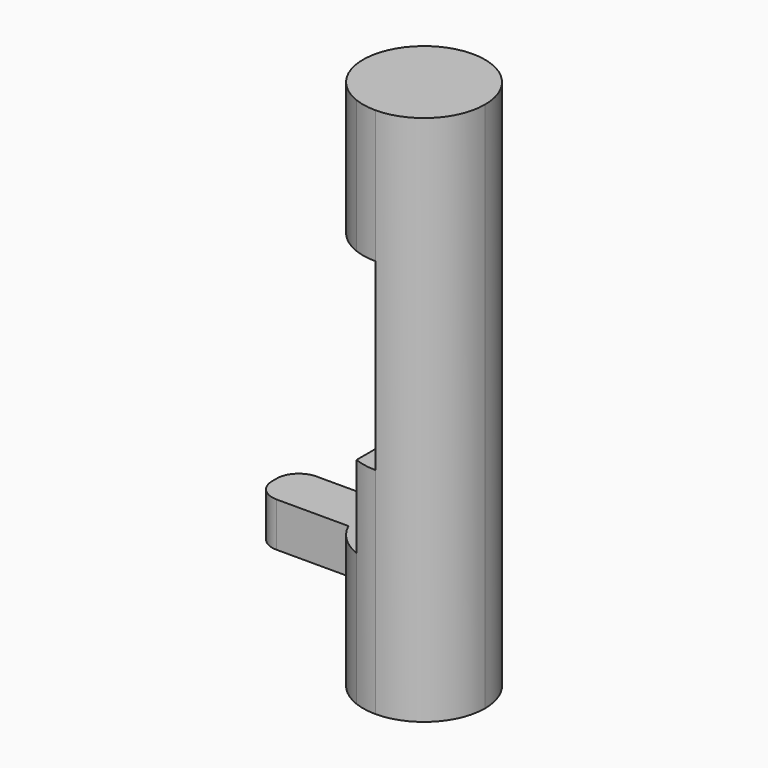
from build123d import *
from build123d import SkipClean  # not in build123d's __all__

# Parameters (mm, degrees)
F1_DEPTH = 24
F2_DEPTH = 18
F3_DEPTH = 9.7
F4_DEPTH = 6
F5_DEPTH = 6
F6_R     = 1
F7_DEPTH = 4


with BuildPart() as f1:
    # F0 (on Top) → F1 (new body)
    with BuildSketch(Plane.XY):
        with BuildLine():
            ThreePointArc((0, -2.75), (1.9445436483, -1.9445436483), (2.75, 0))
            ThreePointArc((2.75, 0), (1.9445436483, 1.9445436483), (0, 2.75))
            Line((0, 2.75), (0, 1.12))
            Line((0, 1.12), (0, 0))
            Line((0, 0), (0, -1.13))
            Line((0, -1.13), (0, -2.75))
        make_face()
        with BuildLine():
            Line((0, 1.12), (0, 2.75))
            ThreePointArc((0, 2.75), (-0.5087835239, 2.7025246208), (-1, 2.5617376915))
            Line((-1, 2.5617376915), (-1, 1.12))
            Line((-1, 1.12), (0, 1.12))
        make_face()
        with BuildLine():
            ThreePointArc((-1, -2.5617376915), (-0.5087835239, -2.7025246208), (0, -2.75))
            Line((0, -2.75), (0, -1.13))
            Line((0, -1.13), (-1, -1.13))
            Line((-1, -1.13), (-1, -2.5617376915))
        make_face()
        with BuildLine():
            Line((-1, 1.12), (-1, 2.5617376915))
            ThreePointArc((-1, 2.5617376915), (-1.8980182962, 1.9899815445), (-2.5115931199, 1.12))
            Line((-2.5115931199, 1.12), (-1, 1.12))
        make_face()
        Polygon((0, 0), (0, 1.12), (-1, 1.12), (-1, -1.13), (0, -1.13), align=None)
        with BuildLine():
            ThreePointArc((-2.5071098899, -1.13), (-1.8940494052, -1.9937594767), (-1, -2.5617376915))
            Line((-1, -2.5617376915), (-1, -1.13))
            Line((-1, -1.13), (-2.5071098899, -1.13))
        make_face()
        with BuildLine():
            Line((-1, 1.12), (-2.5115931199, 1.12))
            ThreePointArc((-2.5115931199, 1.12), (-2.7499945409, -0.0054794925), (-2.5071098899, -1.13))
            Line((-2.5071098899, -1.13), (-1, -1.13))
            Line((-1, -1.13), (-1, 1.12))
        make_face()
    extrude(amount=F1_DEPTH)

    # F0 (on Top) → F2 (cut)
    with BuildSketch(Plane.XY):
        with BuildLine():
            Line((0, 1.12), (0, 2.75))
            ThreePointArc((0, 2.75), (-0.5087835239, 2.7025246208), (-1, 2.5617376915))
            Line((-1, 2.5617376915), (-1, 1.12))
            Line((-1, 1.12), (0, 1.12))
        make_face()
        with BuildLine():
            ThreePointArc((-1, -2.5617376915), (-0.5087835239, -2.7025246208), (0, -2.75))
            Line((0, -2.75), (0, -1.13))
            Line((0, -1.13), (-1, -1.13))
            Line((-1, -1.13), (-1, -2.5617376915))
        make_face()
        with BuildLine():
            Line((-1, 1.12), (-1, 2.5617376915))
            ThreePointArc((-1, 2.5617376915), (-1.8980182962, 1.9899815445), (-2.5115931199, 1.12))
            Line((-2.5115931199, 1.12), (-1, 1.12))
        make_face()
        Polygon((0, 0), (0, 1.12), (-1, 1.12), (-1, -1.13), (0, -1.13), align=None)
        with BuildLine():
            ThreePointArc((-2.5071098899, -1.13), (-1.8940494052, -1.9937594767), (-1, -2.5617376915))
            Line((-1, -2.5617376915), (-1, -1.13))
            Line((-1, -1.13), (-2.5071098899, -1.13))
        make_face()
        with BuildLine():
            Line((-1, 1.12), (-2.5115931199, 1.12))
            ThreePointArc((-2.5115931199, 1.12), (-2.7499945409, -0.0054794925), (-2.5071098899, -1.13))
            Line((-2.5071098899, -1.13), (-1, -1.13))
            Line((-1, -1.13), (-1, 1.12))
        make_face()
    extrude(amount=F2_DEPTH, mode=Mode.SUBTRACT)

    # F0 (on Top) → F3 (join)
    with BuildSketch(Plane.XY):
        with BuildLine():
            Line((0, 1.12), (0, 2.75))
            ThreePointArc((0, 2.75), (-0.5087835239, 2.7025246208), (-1, 2.5617376915))
            Line((-1, 2.5617376915), (-1, 1.12))
            Line((-1, 1.12), (0, 1.12))
        make_face()
        with BuildLine():
            ThreePointArc((-1, -2.5617376915), (-0.5087835239, -2.7025246208), (0, -2.75))
            Line((0, -2.75), (0, -1.13))
            Line((0, -1.13), (-1, -1.13))
            Line((-1, -1.13), (-1, -2.5617376915))
        make_face()
        Polygon((0, 0), (0, 1.12), (-1, 1.12), (-1, -1.13), (0, -1.13), align=None)
    extrude(amount=F3_DEPTH)

    # F0 (on Top) → F4 (join)
    with BuildSketch(Plane.XY):
        with BuildLine():
            Line((-1, 1.12), (-1, 2.5617376915))
            ThreePointArc((-1, 2.5617376915), (-1.8980182962, 1.9899815445), (-2.5115931199, 1.12))
            Line((-2.5115931199, 1.12), (-1, 1.12))
        make_face()
        with BuildLine():
            ThreePointArc((-2.5071098899, -1.13), (-1.8940494052, -1.9937594767), (-1, -2.5617376915))
            Line((-1, -2.5617376915), (-1, -1.13))
            Line((-1, -1.13), (-2.5071098899, -1.13))
        make_face()
        with BuildLine():
            Line((-1, 1.12), (-2.5115931199, 1.12))
            ThreePointArc((-2.5115931199, 1.12), (-2.7499945409, -0.0054794925), (-2.5071098899, -1.13))
            Line((-2.5071098899, -1.13), (-1, -1.13))
            Line((-1, -1.13), (-1, 1.12))
        make_face()
    extrude(amount=F4_DEPTH)

    # F0 (on Top) → F5 (join)
    with BuildSketch(Plane.XY):
        with BuildLine():
            ThreePointArc((-2.5071098899, -1.13), (-2.7499945409, -0.0054794925), (-2.5115931199, 1.12))
            Line((-2.5115931199, 1.12), (-6.75, 1.12))
            Line((-6.75, 1.12), (-6.75, -1.13))
            Line((-6.75, -1.13), (-2.5071098899, -1.13))
        make_face()
    extrude(amount=F5_DEPTH)

    # F6
    f6_edges = [f1.edges().sort_by_distance(p)[0] for p in [
        (-6.75, 1.12, 3),
        (-6.75, -1.13, 3),
    ]]
    fillet(f6_edges, radius=F6_R)

    # F0 (on Top) → F7 (cut)
    with BuildSketch(Plane.XY):
        with BuildLine():
            ThreePointArc((-2.5071098899, -1.13), (-2.7499945409, -0.0054794925), (-2.5115931199, 1.12))
            Line((-2.5115931199, 1.12), (-6.75, 1.12))
            Line((-6.75, 1.12), (-6.75, -1.13))
            Line((-6.75, -1.13), (-2.5071098899, -1.13))
        make_face()
    with SkipClean():  # cleaning this boolean's faces spoils the solid; the shape is the same uncleaned
        extrude(amount=F7_DEPTH, mode=Mode.SUBTRACT)


solid = f1.part
